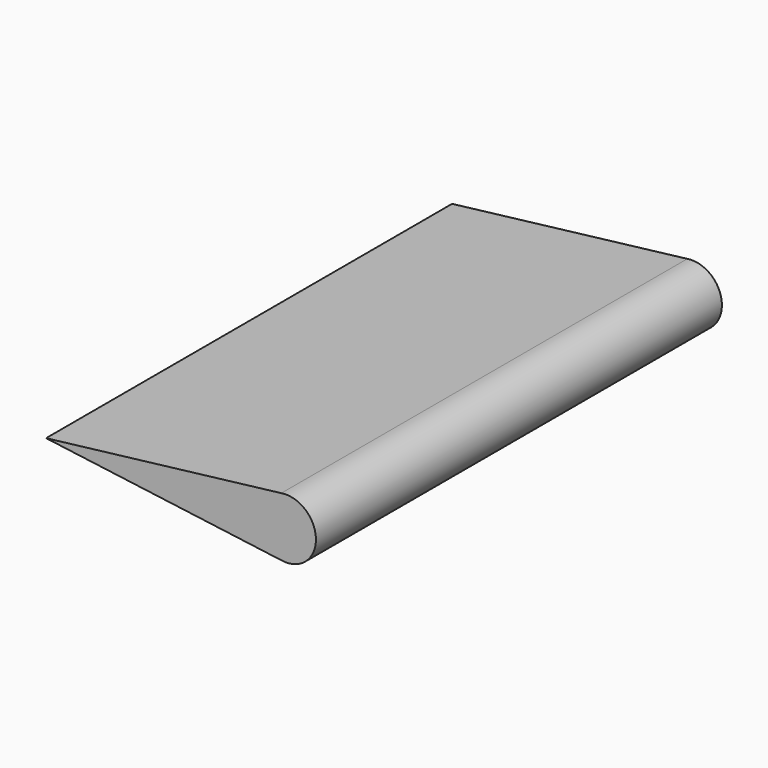
from build123d import *

# Parameters (mm, degrees)
F1_DEPTH = 620.2850937843


# Not quite as in the source:
# - the program builds the solid bodies; features that only make, move or delete a surface that nothing else refers to are left out


with BuildPart() as f1:
    # F0 (on Front) → F1 (new body)
    with BuildSketch(Plane.XZ):
        with BuildLine():
            Line((-287.535071373, 0), (0, -37.9152446985))
            ThreePointArc((0, -37.9152446985), (42.3189124943, -1.8047392368), (0, 34.3057662249))
            Line((0, 34.3057662249), (-287.535071373, 0))
        make_face()
    extrude(amount=F1_DEPTH)


solid = f1.part
